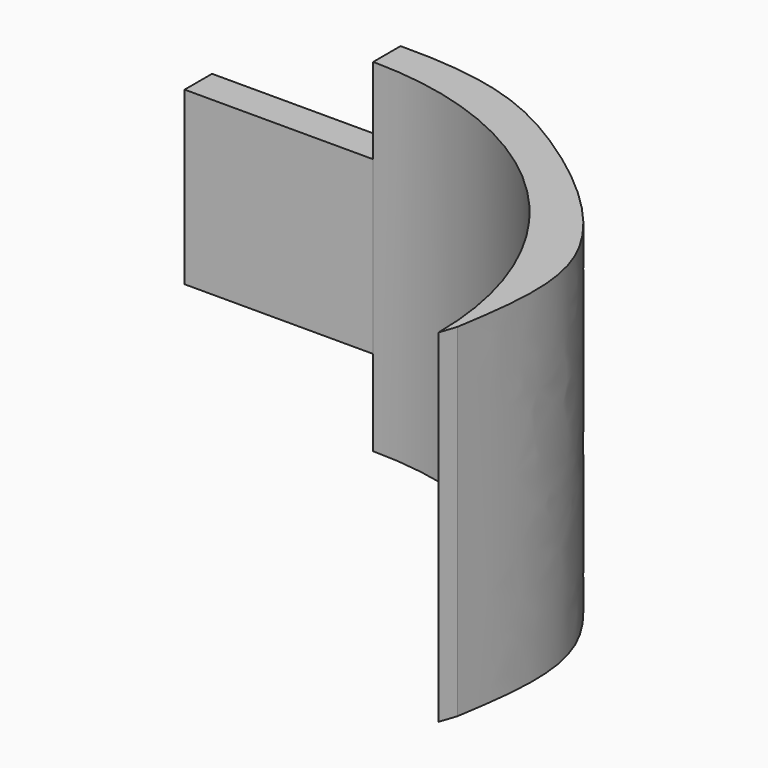
from build123d import *

# Parameters (mm, degrees)
F0_W     = 11
F0_H     = 2
F1_DEPTH = 20
F2_W     = 11
F2_H     = 2
F3_DEPTH = 5
F4_W     = 11
F4_H     = 2
F5_DEPTH = 5


# Not quite as in the source:
# - ends of sketch curves that miss each other by under 0.0002 mm in the source are joined


with BuildPart() as f1:
    # F0 (on Top) → F1 (new body)
    with BuildSketch(Plane.XY):
        with BuildLine():
            ThreePointArc((0, 19), (13.4350288425, 13.4350288425), (19, 0))
            Line((19, 0), (19.3316700079, 0.9884245321))
            add(Edge.make_bspline(
                [(0, 20.9999997169), (5.0418251194, 21.0644266307), (10.6034953843, 19.0446950586), (20.5243171722, 10.6653997718), (19.9493483466, 4.7892186912), (19.3316700079, 0.9884245321)],
                knots=[0, 0, 0, 0, 0.3345544691, 0.6691089382, 0.9528969744, 0.9528969744, 0.9528969744, 0.9528969744], degree=3))
            Line((0, 20.9999997169), (0, 19))
        make_face()
        with Locations((-5.5, 20)):
            Rectangle(F0_W, F0_H)
    extrude(amount=F1_DEPTH)

    # F2 (on face) → F3 (cut)
    with BuildSketch(Plane(origin=(0, 0, 0), x_dir=(1, 0, 0), z_dir=(0, 0, -1))):
        with Locations((-5.5, -20)):
            Rectangle(F2_W, F2_H)
    extrude(amount=-F3_DEPTH, mode=Mode.SUBTRACT)

    # F4 (on face) → F5 (cut)
    with BuildSketch(Plane.XY.offset(20)):
        with Locations((-5.5, 20)):
            Rectangle(F4_W, F4_H)
    extrude(amount=-F5_DEPTH, mode=Mode.SUBTRACT)


solid = f1.part
